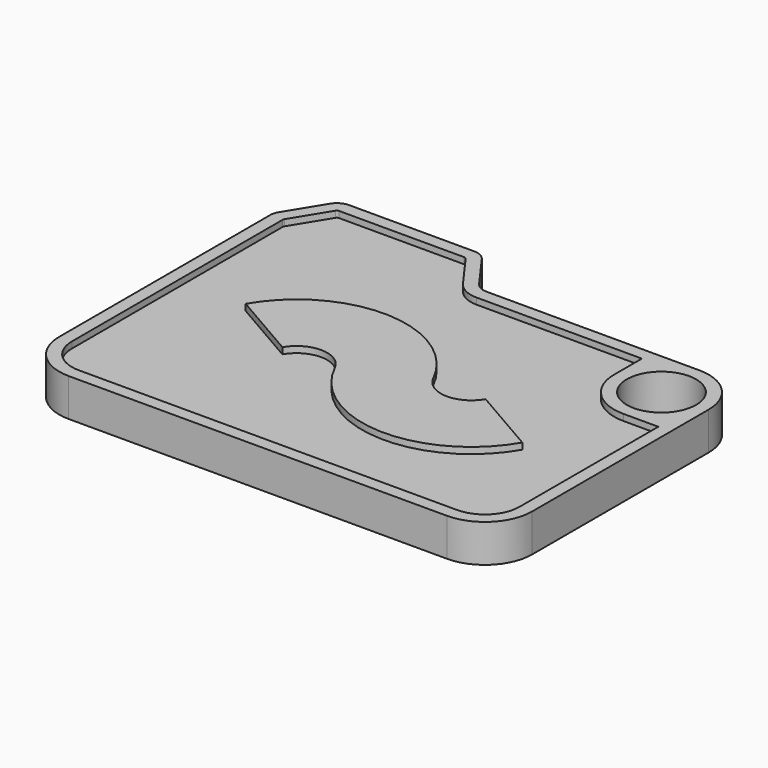
from build123d import *

# Parameters (mm, degrees)
F0_R     = 2.1999998258
F1_DEPTH = 2
F2_DEPTH = 0.4


# Not quite as in the source:
# - ends of sketch curves that miss each other by under 0.0002 mm in the source are joined


with BuildPart() as f1:
    # F0 (on Top) → F1 (new body)
    with BuildSketch(Plane.XY):
        with BuildLine():
            Line((12, 10), (-1.4882636307, 10))
            ThreePointArc((-1.4882636307, 10), (-1.9438159565, 10.1097909917), (-2.2993371991, 10.4150558431))
            Line((-2.2993371991, 10.4150558431), (-3.8642550313, 12.5849441569))
            ThreePointArc((-3.8642550313, 12.5849441569), (-4.2197762739, 12.8902090083), (-4.6753285997, 13))
            Line((-4.6753285997, 13), (-12.6032477109, 13))
            ThreePointArc((-12.6032477109, 13), (-13.0920798627, 12.8723778582), (-13.456140402, 12.5220862548))
            Line((-13.456140402, 12.5220862548), (-14.8528926911, 10.2403180459))
            ThreePointArc((-14.8528926911, 10.2403180459), (-14.9625208286, 9.989439561), (-15, 9.7182317911))
            Line((-15, 9.7182317911), (-15, -7))
            ThreePointArc((-15, -7), (-14.1213203436, -9.1213203436), (-12, -10))
            Line((-12, -10), (12, -10))
            ThreePointArc((12, -10), (14.1213203436, -9.1213203436), (15, -7))
            Line((15, -7), (15, 7))
            ThreePointArc((15, 7), (14.1213203436, 9.1213203436), (12, 10))
        make_face()
        with BuildLine():
            ThreePointArc((-14.1999998258, 9.7182317911), (-14.192503998, 9.7724732978), (-14.1705783896, 9.8226489511))
            Line((-14.1705783896, 9.8226489511), (-12.7738261005, 12.10441716))
            ThreePointArc((-12.7738261005, 12.10441716), (-12.7010140561, 12.1744754196), (-12.6032477109, 12.1999998258))
            Line((-12.6032477109, 12.1999998258), (-4.6753285997, 12.1999998258))
            ThreePointArc((-4.6753285997, 12.1999998258), (-4.5842182139, 12.1780416465), (-4.5131140273, 12.1169887295))
            Line((-4.5131140273, 12.1169887295), (-2.9481961951, 9.9471004156))
            ThreePointArc((-2.9481961951, 9.9471004156), (-2.3082578965, 9.3976236299), (-1.4882636307, 9.1999998258))
            Line((-1.4882636307, 9.1999998258), (9.0000001742, 9.1999998258))
            Line((9.0000001742, 9.1999998258), (9.0000001742, 7))
            ThreePointArc((9.0000001742, 7), (9.8786797797, 4.8786797797), (12, 4.0000001742))
            Line((12, 4.0000001742), (14.1999998258, 4))
            Line((14.1999998258, 4), (14.1999998258, -7))
            ThreePointArc((14.1999998258, -7), (13.5556347954, -8.5556347954), (12, -9.1999998258))
            Line((12, -9.1999998258), (-12, -9.1999998258))
            ThreePointArc((-12, -9.1999998258), (-13.5556347954, -8.5556347954), (-14.1999998258, -7))
            Line((-14.1999998258, -7), (-14.1999998258, 9.7182317911))
        make_face(mode=Mode.SUBTRACT)
        with Locations((12, 7)):
            Circle(F0_R, mode=Mode.SUBTRACT)
        with BuildLine():
            Line((-12.7738261005, 12.10441716), (-14.1705783896, 9.8226489511))
            ThreePointArc((-14.1705783896, 9.8226489511), (-14.192503998, 9.7724732978), (-14.1999998258, 9.7182317911))
            Line((-14.1999998258, 9.7182317911), (-14.1999998258, -7))
            ThreePointArc((-14.1999998258, -7), (-13.5556347954, -8.5556347954), (-12, -9.1999998258))
            Line((-12, -9.1999998258), (12, -9.1999998258))
            ThreePointArc((12, -9.1999998258), (13.5556347954, -8.5556347954), (14.1999998258, -7))
            Line((14.1999998258, -7), (14.1999998258, 4))
            Line((14.1999998258, 4), (12, 4))
            ThreePointArc((12, 4), (9.8786797797, 4.8786797797), (9.0000001742, 7))
            Line((9.0000001742, 7), (9.0000001742, 9.1999998258))
            Line((9.0000001742, 9.1999998258), (-1.4882636307, 9.1999998258))
            ThreePointArc((-1.4882636307, 9.1999998258), (-2.3082578965, 9.3976236299), (-2.9481961951, 9.9471004156))
            Line((-2.9481961951, 9.9471004156), (-4.5131140273, 12.1169887295))
            ThreePointArc((-4.5131140273, 12.1169887295), (-4.5842182139, 12.1780416465), (-4.6753285997, 12.1999998258))
            Line((-4.6753285997, 12.1999998258), (-12.6032477109, 12.1999998258))
            ThreePointArc((-12.6032477109, 12.1999998258), (-12.7010140561, 12.1744754196), (-12.7738261005, 12.10441716))
        make_face()
        with BuildLine():
            ThreePointArc((10, -1.5313274312), (3.7431454959, -4.9955321683), (-2.2491392669, -1.0915001412))
            ThreePointArc((-2.2491392669, -1.0915001412), (-3.9225638289, -0.0012477009), (-5.6698729811, -0.9686725688))
            Line((-5.6698729811, -0.9686725688), (-10, 1.5313274312))
            ThreePointArc((-10, 1.5313274312), (-3.7431454959, 4.9955321683), (2.2491392669, 1.0915001412))
            ThreePointArc((2.2491392669, 1.0915001412), (3.9225638289, 0.0012477009), (5.6698729811, 0.9686725688))
            Line((5.6698729811, 0.9686725688), (10, -1.5313274312))
        make_face(mode=Mode.SUBTRACT)
        with BuildLine():
            ThreePointArc((-5.6698729811, -0.9686725688), (-3.9225638289, -0.0012477009), (-2.2491392669, -1.0915001412))
            ThreePointArc((-2.2491392669, -1.0915001412), (3.7431454959, -4.9955321683), (10, -1.5313274312))
            Line((10, -1.5313274312), (5.6698729811, 0.9686725688))
            ThreePointArc((5.6698729811, 0.9686725688), (3.9225638289, 0.0012477009), (2.2491392669, 1.0915001412))
            ThreePointArc((2.2491392669, 1.0915001412), (-3.7431454959, 4.9955321683), (-10, 1.5313274312))
            Line((-10, 1.5313274312), (-5.6698729811, -0.9686725688))
        make_face()
    extrude(amount=-F1_DEPTH)

    # F0 (on Top) → F2 (join)
    with BuildSketch(Plane.XY):
        with BuildLine():
            Line((12, 10), (-1.4882636307, 10))
            ThreePointArc((-1.4882636307, 10), (-1.9438159565, 10.1097909917), (-2.2993371991, 10.4150558431))
            Line((-2.2993371991, 10.4150558431), (-3.8642550313, 12.5849441569))
            ThreePointArc((-3.8642550313, 12.5849441569), (-4.2197762739, 12.8902090083), (-4.6753285997, 13))
            Line((-4.6753285997, 13), (-12.6032477109, 13))
            ThreePointArc((-12.6032477109, 13), (-13.0920798627, 12.8723778582), (-13.456140402, 12.5220862548))
            Line((-13.456140402, 12.5220862548), (-14.8528926911, 10.2403180459))
            ThreePointArc((-14.8528926911, 10.2403180459), (-14.9625208286, 9.989439561), (-15, 9.7182317911))
            Line((-15, 9.7182317911), (-15, -7))
            ThreePointArc((-15, -7), (-14.1213203436, -9.1213203436), (-12, -10))
            Line((-12, -10), (12, -10))
            ThreePointArc((12, -10), (14.1213203436, -9.1213203436), (15, -7))
            Line((15, -7), (15, 7))
            ThreePointArc((15, 7), (14.1213203436, 9.1213203436), (12, 10))
        make_face()
        with BuildLine():
            ThreePointArc((-14.1999998258, 9.7182317911), (-14.192503998, 9.7724732978), (-14.1705783896, 9.8226489511))
            Line((-14.1705783896, 9.8226489511), (-12.7738261005, 12.10441716))
            ThreePointArc((-12.7738261005, 12.10441716), (-12.7010140561, 12.1744754196), (-12.6032477109, 12.1999998258))
            Line((-12.6032477109, 12.1999998258), (-4.6753285997, 12.1999998258))
            ThreePointArc((-4.6753285997, 12.1999998258), (-4.5842182139, 12.1780416465), (-4.5131140273, 12.1169887295))
            Line((-4.5131140273, 12.1169887295), (-2.9481961951, 9.9471004156))
            ThreePointArc((-2.9481961951, 9.9471004156), (-2.3082578965, 9.3976236299), (-1.4882636307, 9.1999998258))
            Line((-1.4882636307, 9.1999998258), (9.0000001742, 9.1999998258))
            Line((9.0000001742, 9.1999998258), (9.0000001742, 7))
            ThreePointArc((9.0000001742, 7), (9.8786797797, 4.8786797797), (12, 4.0000001742))
            Line((12, 4.0000001742), (14.1999998258, 4))
            Line((14.1999998258, 4), (14.1999998258, -7))
            ThreePointArc((14.1999998258, -7), (13.5556347954, -8.5556347954), (12, -9.1999998258))
            Line((12, -9.1999998258), (-12, -9.1999998258))
            ThreePointArc((-12, -9.1999998258), (-13.5556347954, -8.5556347954), (-14.1999998258, -7))
            Line((-14.1999998258, -7), (-14.1999998258, 9.7182317911))
        make_face(mode=Mode.SUBTRACT)
        with Locations((12, 7)):
            Circle(F0_R, mode=Mode.SUBTRACT)
        with BuildLine():
            ThreePointArc((-5.6698729811, -0.9686725688), (-3.9225638289, -0.0012477009), (-2.2491392669, -1.0915001412))
            ThreePointArc((-2.2491392669, -1.0915001412), (3.7431454959, -4.9955321683), (10, -1.5313274312))
            Line((10, -1.5313274312), (5.6698729811, 0.9686725688))
            ThreePointArc((5.6698729811, 0.9686725688), (3.9225638289, 0.0012477009), (2.2491392669, 1.0915001412))
            ThreePointArc((2.2491392669, 1.0915001412), (-3.7431454959, 4.9955321683), (-10, 1.5313274312))
            Line((-10, 1.5313274312), (-5.6698729811, -0.9686725688))
        make_face()
    extrude(amount=F2_DEPTH)


solid = f1.part
